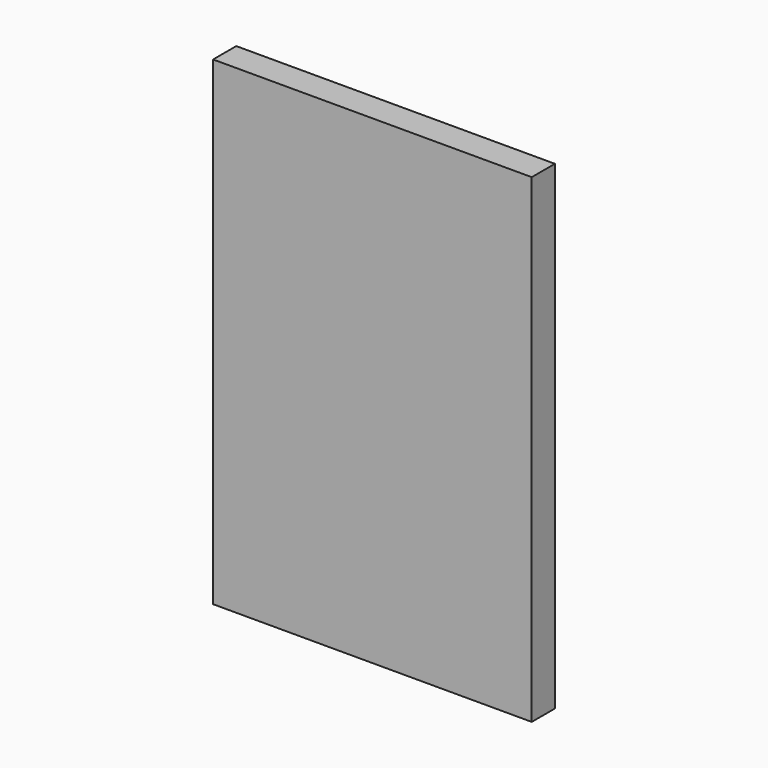
from build123d import *

# Parameters (mm, degrees)
F0_W     = 198
F0_H     = 298
F1_DEPTH = 18


# Not quite as in the source:
# - a feature names something its author has since deleted; it is built from what else it names


with BuildPart() as f1:
    # F0 (on Front) → F1 (new body)
    with BuildSketch(Plane.XZ):
        Rectangle(F0_W, F0_H)
    extrude(amount=F1_DEPTH)


solid = f1.part
